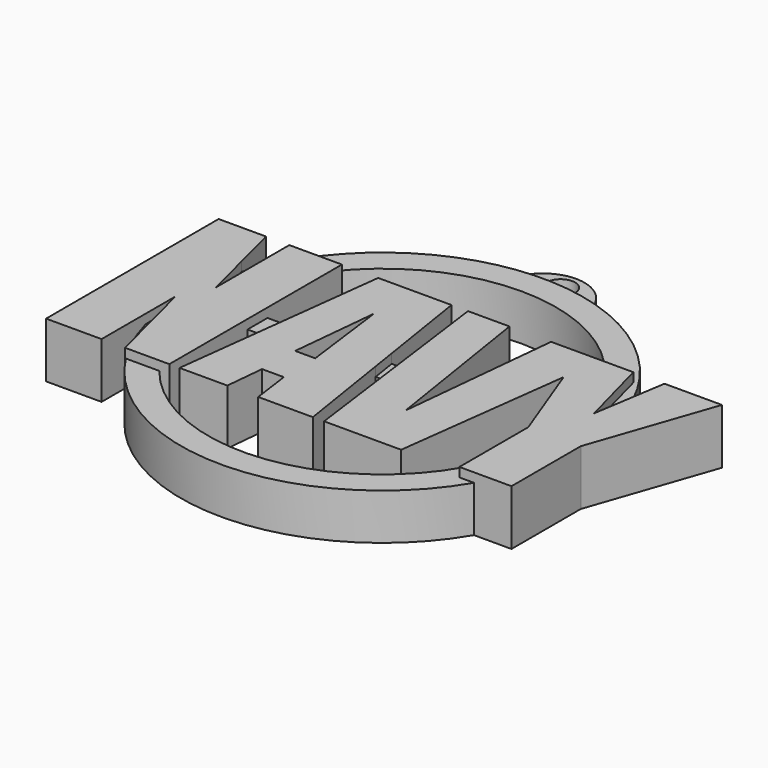
from build123d import *

# Parameters (mm, degrees)
F1_DEPTH = 6.096
F2_DEPTH = 5.08
F0_R     = 1.5875
F3_DEPTH = 3.175
F4_DEPTH = 5.08


# Not quite as in the source:
# - a feature names something its author has since deleted; it is built from what else it names


with BuildPart() as f1:
    # F0 (on Top) → F1 (new body)
    with BuildSketch(Plane.XY):
        Polygon((-24.1886169598, 3.2886979016), (-29.4082708062, 3.2886979016), (-29.4082708062, -20.4897223923), (-23.292648052, -20.4897223923), (-23.292648052, -14.4124455645), (-23.292648052, -10.3212194436), (-20.7735943805, -20.2349212979), (-20.7088498843, -20.4897223923), (-20.6143816365, -20.4897223923), (-16.92762383, -20.4897223923), (-15.8206042222, -20.4897223923), (-15.8206042222, -9.7183147231), (-15.8206042222, -6.9649312645), (-15.8206042222, 3.2886979016), (-16.92762383, 3.2886979016), (-20.6143816365, 3.2886979016), (-21.6202178109, 3.2886979016), (-21.6202178109, 1.5303949543), (-21.6202178109, -6.8192024151), (-22.9411163325, -1.6208240435), align=None)
    extrude(amount=F1_DEPTH)



with BuildPart() as f1b:
    # F0 (on Top) → F1, piece 2 (new body)
    with BuildSketch(Plane.XY):
        Polygon((-11.8259407802, 3.2886979016), (-13.0638151335, -6.9649312645), (-13.3962186866, -9.7183147231), (-14.6966021007, -20.4897223923), (-9.4239554059, -20.4897223923), (-9.0138624712, -16.2260920352), (-6.6118787134, -16.2260920352), (-6.0260297393, -20.4897223923), (0, -20.4897223923), (-1.6947368922, -9.7183147231), (-2.1279449434, -6.9649312645), (-3.7412163152, 3.2886979016), align=None)
        Polygon((-8.9032554867, -11.7976386267), (-7.9436938241, -2.1282115334), (-6.6930804921, -11.7976386267), align=None, mode=Mode.SUBTRACT)
    extrude(amount=F1_DEPTH)


with BuildPart() as f1c:
    # F0 (on Top) → F1, piece 3 (new body)
    with BuildSketch(Plane.XY):
        Polygon((16.3027588278, 3.2886979016), (13.1864075148, 3.2886979016), (7.2406129912, 3.2886979016), (5.4566214701, -14.5271265076), (2.6535398471, 3.2886979016), (-1.9227857701, 3.2886979016), (-0.5595875609, -6.9649312645), (-0.1935310809, -9.7183147231), (1.23850468, -20.4897223923), (9.7333230228, -20.4897223923), (12.1938914085, -1.1697572338), (15.6504033197, -10.3675947497), (15.6504033197, -16.4159582139), (15.6504033197, -19.8583583692), (17.259035404, -19.8583583692), (21.3917291938, -19.8583583692), (21.3917291938, -10.3090095828), (26.0736756027, 3.2886979016), (19.7453610599, 3.2886979016), (19.0404757801, -1.1567947134), (18.4624816288, -4.8020243761), align=None)
    extrude(amount=F1_DEPTH)


with BuildPart() as f1_1:
    add(f1.part)

    add(f1c.part)  # F2 merges F1c
    # F0 (on Top) → F2 (join)
    with BuildSketch(Plane.XY):
        with BuildLine():
            ThreePointArc((-6.4941192245, 13.1090595505), (-14.544099093, 9.6221382111), (-20.6143816365, 3.2886979016))
            Line((-20.6143816365, 3.2886979016), (-16.92762383, 3.2886979016))
            ThreePointArc((-16.92762383, 3.2886979016), (-1.8706081576, 10.5845610899), (13.1864075148, 3.2886979016))
            Line((13.1864075148, 3.2886979016), (16.3027588278, 3.2886979016))
            Line((16.3027588278, 3.2886979016), (18.4624816288, -4.8020243761))
            Line((18.4624816288, -4.8020243761), (19.0404757801, -1.1567947134))
            ThreePointArc((19.0404757801, -1.1567947134), (12.7148241923, 8.1311202307), (2.6507858926, 13.130556711))
            ThreePointArc((2.6507858926, 13.130556711), (-1.9227857701, 13.595875741), (-6.4941192245, 13.1090595505))
        make_face()
        with BuildLine():
            ThreePointArc((-21.6202178109, 1.5303949543), (-22.3413934423, -0.0197598322), (-22.9411163325, -1.6208240435))
            Line((-22.9411163325, -1.6208240435), (-21.6202178109, -6.8192024151))
            Line((-21.6202178109, -6.8192024151), (-21.6202178109, 1.5303949543))
        make_face()
        with BuildLine():
            Line((-23.292648052, -10.3212194436), (-23.292648052, -14.4124455645))
            ThreePointArc((-23.292648052, -14.4124455645), (-22.2422118931, -17.4141450598), (-20.7735943805, -20.2349212979))
            Line((-20.7735943805, -20.2349212979), (-23.292648052, -10.3212194436))
        make_face()
        with BuildLine():
            Line((-16.92762383, -20.4897223923), (-20.6143816365, -20.4897223923))
            ThreePointArc((-20.6143816365, -20.4897223923), (-1.5006364525, -30.7938779901), (17.259035404, -19.8583583692))
            Line((17.259035404, -19.8583583692), (15.6504033197, -19.8583583692))
            Line((15.6504033197, -19.8583583692), (15.6504033197, -16.4159582139))
            ThreePointArc((15.6504033197, -16.4159582139), (0.5098765571, -27.6373274044), (-16.92762383, -20.4897223923))
        make_face()
    extrude(amount=F2_DEPTH)

    # F0 (on Top) → F3 (join)
    with BuildSketch(Plane.XY):
        with BuildLine():
            ThreePointArc((2.6507858926, 13.130556711), (-1.933592452, 18.1930447362), (-6.4941192245, 13.1090595505))
            ThreePointArc((-6.4941192245, 13.1090595505), (-1.9227857701, 13.595875741), (2.6507858926, 13.130556711))
        make_face()
        with Locations((-1.9227857701, 16.0606782883)):
            Circle(F0_R, mode=Mode.SUBTRACT)
    extrude(amount=F3_DEPTH)


    add(f1b.part)  # F4 merges F1b
    # F0 (on Top) → F4 (join)
    with BuildSketch(Plane.XY):
        Polygon((-13.0638151335, -6.9649312645), (-15.8206042222, -6.9649312645), (-15.8206042222, -9.7183147231), (-13.3962186866, -9.7183147231), align=None)
        Polygon((-0.5595875609, -6.9649312645), (-2.1279449434, -6.9649312645), (-1.6947368922, -9.7183147231), (-0.1935310809, -9.7183147231), align=None)
    extrude(amount=F4_DEPTH)


solid = f1_1.part
